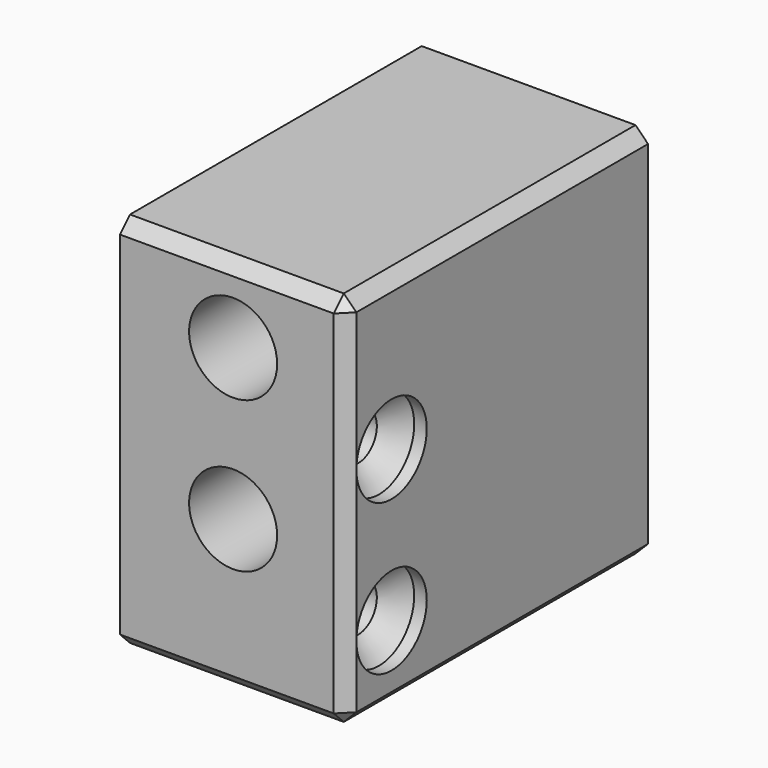
from build123d import *

# Parameters (mm, degrees)
F0_W           = 18
F0_H           = 30
F1_DEPTH       = 30
F4_D           = 7
F4_DEPTH       = 15.001
F5_D           = 3.7
F5_CSINK_D     = 7
F5_CSINK_ANGLE = 90
F8_D           = 7
F8_DEPTH       = 1.001
F9_D           = 3.7
F9_CSINK_D     = 7
F9_CSINK_ANGLE = 90
F10_SIZE       = 0.99999


# Not quite as in the source:
# - a fillet or chamfer is up to 0.001 mm smaller than in the source, because OpenCascade refuses the exact size


with BuildPart() as f1:
    # F0 (on Front) → F1 (new body)
    with BuildSketch(Plane.XZ):
        with Locations((0, 15)):
            Rectangle(F0_W, F0_H)
    extrude(amount=F1_DEPTH)

    # F4 (through all, one way)
    with BuildSketch(Plane(origin=(0, -15, 0), x_dir=(1, 0, 0), z_dir=(0, 1, 0))):
        with Locations((0, -24), (0, -12)):
            Circle(F4_D / 2)
    extrude(amount=-F4_DEPTH, mode=Mode.SUBTRACT)

    # F5 (through all)
    with Locations(Plane.XZ.offset(15)):
        with Locations((0, 24), (0, 12)):
            CounterSinkHole(F5_D / 2, F5_CSINK_D / 2, counter_sink_angle=F5_CSINK_ANGLE)

    # F8 (through all, one way)
    with BuildSketch(Plane(origin=(8, 0, 0), x_dir=(0, 1, 0), z_dir=(-1, 0, 0))):
        with Locations((-25.5, -18), (-25.5, -6)):
            Circle(F8_D / 2)
    extrude(amount=-F8_DEPTH, mode=Mode.SUBTRACT)

    # F9 (through all)
    with Locations(Plane.YZ.offset(8)):
        with Locations((-25.5, 18), (-25.5, 6)):
            CounterSinkHole(F9_D / 2, F9_CSINK_D / 2, counter_sink_angle=F9_CSINK_ANGLE)

    # F10 (size 1 in the source; OpenCascade refuses exactly that, so slightly less here)
    f10_edges = [f1.edges().sort_by_distance(p)[0] for p in [
        (9, -30, 15),
        (9, -15, 30),
        (0, -30, 30),
        (9, -15, 0),
        (0, -30, 0),
    ]]
    chamfer(f10_edges, length=F10_SIZE)


solid = f1.part
